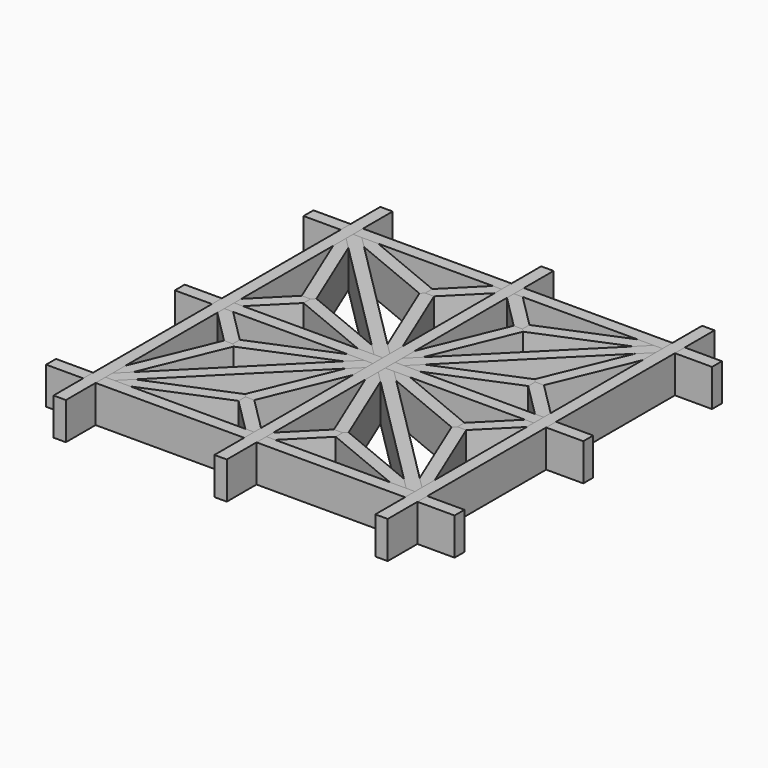
from build123d import *

# Parameters (mm, degrees)
F0_W      = 3.175
F0_H      = 104.775
F1_DEPTH  = 9.525
F2_W      = 3.175
F2_H      = 4.7625
F3_DEPTH  = 85.726
F4_W      = 104.775
F4_H      = 3.175
F5_DEPTH  = 4.7625
F6_W      = 38.1
F6_H      = 3.175
F6_W_2    = 9.525
F7_DEPTH  = 4.7625
F9_DEPTH  = 9.525
F11_DEPTH = 9.525
F12_DEPTH = 9.525
F13_DEPTH = 9.525


with BuildPart() as f1:
    # F0 (on Top) → F1 (new body)
    with BuildSketch(Plane.XY):
        with Locations((1.5875, -52.3875)):
            Rectangle(F0_W, F0_H)
    extrude(amount=F1_DEPTH)


with BuildPart() as f1b:
    # F0 (on Top) → F1, piece 2 (new body)
    with BuildSketch(Plane.XY):
        with Locations((42.8625, -52.3875)):
            Rectangle(F0_W, F0_H)
    extrude(amount=F1_DEPTH)


with BuildPart() as f1c:
    # F0 (on Top) → F1, piece 3 (new body)
    with BuildSketch(Plane.XY):
        with Locations((84.1375, -52.3875)):
            Rectangle(F0_W, F0_H)
    extrude(amount=F1_DEPTH)


with BuildPart() as f3_tool:
    # F2 (on face) → F3 (new body, through all)
    with BuildSketch(Plane.YZ.offset(85.725)):
        with Locations((-93.6625, 2.38125)):
            Rectangle(F2_W, F2_H)
        with Locations((-52.3875, 2.38125)):
            Rectangle(F2_W, F2_H)
        with Locations((-11.1125, 2.38125)):
            Rectangle(F2_W, F2_H)
    extrude(amount=-F3_DEPTH)


with BuildPart() as f1_1:
    add(f1.part)

    # F3: cut by f3_tool
    add(f3_tool.part, mode=Mode.SUBTRACT)


with BuildPart() as f1b_1:
    add(f1b.part)

    # F3: cut by f3_tool
    add(f3_tool.part, mode=Mode.SUBTRACT)


with BuildPart() as f1c_1:
    add(f1c.part)

    # F3: cut by f3_tool
    add(f3_tool.part, mode=Mode.SUBTRACT)


with BuildPart() as f5:
    # F4 (on Top) → F5 (new body, through all)
    with BuildSketch(Plane.XY):
        with Locations((42.8625, -11.1125)):
            Rectangle(F4_W, F4_H)
    extrude(amount=F5_DEPTH)

    # F6 (on face) → F7, piece 3 (join, through all)
    with BuildSketch(Plane.XY.offset(4.7625)):
        with Locations((22.225, -11.1125)):
            Rectangle(F6_W, F6_H)
        with Locations((63.5, -11.1125)):
            Rectangle(F6_W, F6_H)
        with Locations((90.4875, -11.1125)):
            Rectangle(F6_W_2, F6_H)
        with Locations((-4.7625, -11.1125)):
            Rectangle(F6_W_2, F6_H)
    extrude(amount=F7_DEPTH)


with BuildPart() as f5b:
    # F4 (on Top) → F5, piece 2 (new body, through all)
    with BuildSketch(Plane.XY):
        with Locations((42.8625, -52.3875)):
            Rectangle(F4_W, F4_H)
    extrude(amount=F5_DEPTH)

    # F6 (on face) → F7, piece 2 (join, through all)
    with BuildSketch(Plane.XY.offset(4.7625)):
        with Locations((22.225, -52.3875)):
            Rectangle(F6_W, F6_H)
        with Locations((63.5, -52.3875)):
            Rectangle(F6_W, F6_H)
        with Locations((90.4875, -52.3875)):
            Rectangle(F6_W_2, F6_H)
        with Locations((-4.7625, -52.3875)):
            Rectangle(F6_W_2, F6_H)
    extrude(amount=F7_DEPTH)


with BuildPart() as f5c:
    # F4 (on Top) → F5, piece 3 (new body, through all)
    with BuildSketch(Plane.XY):
        with Locations((42.8625, -93.6625)):
            Rectangle(F4_W, F4_H)
    extrude(amount=F5_DEPTH)

    # F6 (on face) → F7 (join, through all)
    with BuildSketch(Plane.XY.offset(4.7625)):
        with Locations((22.225, -93.6625)):
            Rectangle(F6_W, F6_H)
        with Locations((63.5, -93.6625)):
            Rectangle(F6_W, F6_H)
        with Locations((90.4875, -93.6625)):
            Rectangle(F6_W_2, F6_H)
        with Locations((-4.7625, -93.6625)):
            Rectangle(F6_W_2, F6_H)
    extrude(amount=F7_DEPTH)


with BuildPart() as f9:
    # F8 (on Top) → F9 (new body, through all)
    with BuildSketch(Plane.XY):
        Polygon((82.55, -89.8299359697), (46.6950640303, -53.975), (44.45, -53.975), (44.45, -56.2200640303), (80.3049359697, -92.075), (82.55, -92.075), align=None)
    extrude(amount=F9_DEPTH)


with BuildPart() as f9b:
    # F8 (on Top) → F9, piece 2 (new body, through all)
    with BuildSketch(Plane.XY):
        Polygon((46.6950640303, -50.8), (82.55, -14.9450640303), (82.55, -12.7), (80.3049359697, -12.7), (44.45, -48.5549359697), (44.45, -50.8), align=None)
    extrude(amount=F9_DEPTH)


with BuildPart() as f9c:
    # F8 (on Top) → F9, piece 3 (new body, through all)
    with BuildSketch(Plane.XY):
        Polygon((39.0299359697, -50.8), (41.275, -50.8), (41.275, -48.5549359697), (5.4200640303, -12.7), (3.175, -12.7), (3.175, -14.9450640303), align=None)
    extrude(amount=F9_DEPTH)


with BuildPart() as f9d:
    # F8 (on Top) → F9, piece 4 (new body, through all)
    with BuildSketch(Plane.XY):
        Polygon((5.4200640303, -92.075), (41.275, -56.2200640303), (41.275, -53.975), (39.0299359697, -53.975), (3.175, -89.8299359697), (3.175, -92.075), align=None)
    extrude(amount=F9_DEPTH)


with BuildPart() as f11:
    # F10 (on Top) → F11 (new body, through all)
    with BuildSketch(Plane.XY):
        Polygon((76.1565985563, -12.7), (55.3241477088, -21.3290836785), (55.3241477088, -23.5741477088), (56.1666875043, -24.4166875043), (77.371618454, -15.6333175157), (80.3049359697, -12.7), align=None)
    extrude(amount=F11_DEPTH)


with BuildPart() as f11b:
    # F10 (on Top) → F11, piece 2 (new body, through all)
    with BuildSketch(Plane.XY):
        Polygon((71.6758522912, -39.9258522912), (73.9209163215, -39.9258522912), (82.55, -19.0934014437), (82.55, -14.9450640303), (79.6166824843, -17.878381546), (70.8333124957, -39.0833124957), align=None)
    extrude(amount=F11_DEPTH)


with BuildPart() as f11c:
    # F10 (on Top) → F11, piece 3 (new body, through all)
    with BuildSketch(Plane.XY):
        Polygon((73.9209163215, -64.8491477088), (71.6758522912, -64.8491477088), (70.8333124957, -65.6916875043), (79.6166824843, -86.896618454), (82.55, -89.8299359697), (82.55, -85.6815985563), align=None)
    extrude(amount=F11_DEPTH)


with BuildPart() as f11d:
    # F10 (on Top) → F11, piece 4 (new body, through all)
    with BuildSketch(Plane.XY):
        Polygon((77.371618454, -89.1416824843), (56.1666875043, -80.3583124957), (55.3241477088, -81.2008522912), (55.3241477088, -83.4459163215), (76.1565985563, -92.075), (80.3049359697, -92.075), align=None)
    extrude(amount=F11_DEPTH)


with BuildPart() as f11e:
    # F10 (on Top) → F11, piece 5 (new body, through all)
    with BuildSketch(Plane.XY):
        Polygon((30.4008522912, -83.4459163215), (30.4008522912, -81.2008522912), (29.5583124957, -80.3583124957), (8.353381546, -89.1416824843), (5.4200640303, -92.075), (9.5684014437, -92.075), align=None)
    extrude(amount=F11_DEPTH)


with BuildPart() as f11f:
    # F10 (on Top) → F11, piece 6 (new body, through all)
    with BuildSketch(Plane.XY):
        Polygon((14.8916875043, -65.6916875043), (14.0491477088, -64.8491477088), (11.8040836785, -64.8491477088), (3.175, -85.6815985563), (3.175, -89.8299359697), (6.1083175157, -86.896618454), align=None)
    extrude(amount=F11_DEPTH)


with BuildPart() as f11g:
    # F10 (on Top) → F11, piece 7 (new body, through all)
    with BuildSketch(Plane.XY):
        Polygon((3.175, -14.9450640303), (3.175, -19.0934014437), (11.8040836785, -39.9258522912), (14.0491477088, -39.9258522912), (14.8916875043, -39.0833124957), (6.1083175157, -17.878381546), align=None)
    extrude(amount=F11_DEPTH)


with BuildPart() as f11h:
    # F10 (on Top) → F11, piece 8 (new body, through all)
    with BuildSketch(Plane.XY):
        Polygon((30.4008522912, -23.5741477088), (30.4008522912, -21.3290836785), (9.5684014437, -12.7), (5.4200640303, -12.7), (8.353381546, -15.6333175157), (29.5583124957, -24.4166875043), align=None)
    extrude(amount=F11_DEPTH)


with BuildPart() as f12:
    # F10 (on Top) → F12 (new body, through all)
    with BuildSketch(Plane.XY):
        Polygon((56.1666875043, -24.4166875043), (55.3241477088, -23.5741477088), (53.0790836785, -23.5741477088), (44.45, -44.4065985563), (44.45, -48.5549359697), (47.3833175157, -45.621618454), align=None)
    extrude(amount=F12_DEPTH)


with BuildPart() as f12b:
    # F10 (on Top) → F12, piece 2 (new body, through all)
    with BuildSketch(Plane.XY):
        Polygon((71.6758522912, -42.1709163215), (71.6758522912, -39.9258522912), (70.8333124957, -39.0833124957), (49.628381546, -47.8666824843), (46.6950640303, -50.8), (50.8434014437, -50.8), align=None)
    extrude(amount=F12_DEPTH)


with BuildPart() as f12c:
    # F10 (on Top) → F12, piece 3 (new body, through all)
    with BuildSketch(Plane.XY):
        Polygon((71.6758522912, -64.8491477088), (71.6758522912, -62.6040836785), (50.8434014437, -53.975), (46.6950640303, -53.975), (49.628381546, -56.9083175157), (70.8333124957, -65.6916875043), align=None)
    extrude(amount=F12_DEPTH)


with BuildPart() as f12d:
    # F10 (on Top) → F12, piece 4 (new body, through all)
    with BuildSketch(Plane.XY):
        Polygon((47.3833175157, -59.153381546), (44.45, -56.2200640303), (44.45, -60.3684014437), (53.0790836785, -81.2008522912), (55.3241477088, -81.2008522912), (56.1666875043, -80.3583124957), align=None)
    extrude(amount=F12_DEPTH)


with BuildPart() as f12e:
    # F10 (on Top) → F12, piece 5 (new body, through all)
    with BuildSketch(Plane.XY):
        Polygon((30.4008522912, -81.2008522912), (32.6459163215, -81.2008522912), (41.275, -60.3684014437), (41.275, -56.2200640303), (38.3416824843, -59.153381546), (29.5583124957, -80.3583124957), align=None)
    extrude(amount=F12_DEPTH)


with BuildPart() as f12f:
    # F10 (on Top) → F12, piece 6 (new body, through all)
    with BuildSketch(Plane.XY):
        Polygon((34.8815985563, -53.975), (14.0491477088, -62.6040836785), (14.0491477088, -64.8491477088), (14.8916875043, -65.6916875043), (36.096618454, -56.9083175157), (39.0299359697, -53.975), align=None)
    extrude(amount=F12_DEPTH)


with BuildPart() as f12g:
    # F10 (on Top) → F12, piece 7 (new body, through all)
    with BuildSketch(Plane.XY):
        Polygon((14.8916875043, -39.0833124957), (14.0491477088, -39.9258522912), (14.0491477088, -42.1709163215), (34.8815985563, -50.8), (39.0299359697, -50.8), (36.096618454, -47.8666824843), align=None)
    extrude(amount=F12_DEPTH)


with BuildPart() as f12h:
    # F10 (on Top) → F12, piece 8 (new body, through all)
    with BuildSketch(Plane.XY):
        Polygon((41.275, -44.4065985563), (32.6459163215, -23.5741477088), (30.4008522912, -23.5741477088), (29.5583124957, -24.4166875043), (38.3416824843, -45.621618454), (41.275, -48.5549359697), align=None)
    extrude(amount=F12_DEPTH)


with BuildPart() as f13:
    # F10 (on Top) → F13 (new body, through all)
    with BuildSketch(Plane.XY):
        Polygon((55.3241477088, -21.3290836785), (46.6950640303, -12.7), (44.45, -12.7), (44.45, -14.9450640303), (53.0790836785, -23.5741477088), (55.3241477088, -23.5741477088), align=None)
    extrude(amount=F13_DEPTH)


with BuildPart() as f13b:
    # F10 (on Top) → F13, piece 2 (new body, through all)
    with BuildSketch(Plane.XY):
        Polygon((82.55, -48.5549359697), (73.9209163215, -39.9258522912), (71.6758522912, -39.9258522912), (71.6758522912, -42.1709163215), (80.3049359697, -50.8), (82.55, -50.8), align=None)
    extrude(amount=F13_DEPTH)


with BuildPart() as f13c:
    # F10 (on Top) → F13, piece 3 (new body, through all)
    with BuildSketch(Plane.XY):
        Polygon((82.55, -53.975), (80.3049359697, -53.975), (71.6758522912, -62.6040836785), (71.6758522912, -64.8491477088), (73.9209163215, -64.8491477088), (82.55, -56.2200640303), align=None)
    extrude(amount=F13_DEPTH)


with BuildPart() as f13d:
    # F10 (on Top) → F13, piece 4 (new body, through all)
    with BuildSketch(Plane.XY):
        Polygon((55.3241477088, -81.2008522912), (53.0790836785, -81.2008522912), (44.45, -89.8299359697), (44.45, -92.075), (46.6950640303, -92.075), (55.3241477088, -83.4459163215), align=None)
    extrude(amount=F13_DEPTH)


with BuildPart() as f13e:
    # F10 (on Top) → F13, piece 5 (new body, through all)
    with BuildSketch(Plane.XY):
        Polygon((41.275, -89.8299359697), (32.6459163215, -81.2008522912), (30.4008522912, -81.2008522912), (30.4008522912, -83.4459163215), (39.0299359697, -92.075), (41.275, -92.075), align=None)
    extrude(amount=F13_DEPTH)


with BuildPart() as f13f:
    # F10 (on Top) → F13, piece 6 (new body, through all)
    with BuildSketch(Plane.XY):
        Polygon((14.0491477088, -62.6040836785), (5.4200640303, -53.975), (3.175, -53.975), (3.175, -56.2200640303), (11.8040836785, -64.8491477088), (14.0491477088, -64.8491477088), align=None)
    extrude(amount=F13_DEPTH)


with BuildPart() as f13g:
    # F10 (on Top) → F13, piece 7 (new body, through all)
    with BuildSketch(Plane.XY):
        Polygon((14.0491477088, -39.9258522912), (11.8040836785, -39.9258522912), (3.175, -48.5549359697), (3.175, -50.8), (5.4200640303, -50.8), (14.0491477088, -42.1709163215), align=None)
    extrude(amount=F13_DEPTH)


with BuildPart() as f13h:
    # F10 (on Top) → F13, piece 8 (new body, through all)
    with BuildSketch(Plane.XY):
        Polygon((41.275, -14.9450640303), (41.275, -12.7), (39.0299359697, -12.7), (30.4008522912, -21.3290836785), (30.4008522912, -23.5741477088), (32.6459163215, -23.5741477088), align=None)
    extrude(amount=F13_DEPTH)


solid = Compound([f1_1.part, f1b_1.part, f1c_1.part, f5.part, f5b.part, f5c.part, f9.part, f9b.part, f9c.part, f9d.part, f11.part, f11b.part, f11c.part, f11d.part, f11e.part, f11f.part, f11g.part, f11h.part, f12.part, f12b.part, f12c.part, f12d.part, f12e.part, f12f.part, f12g.part, f12h.part, f13.part, f13b.part, f13c.part, f13d.part, f13e.part, f13f.part, f13g.part, f13h.part])
